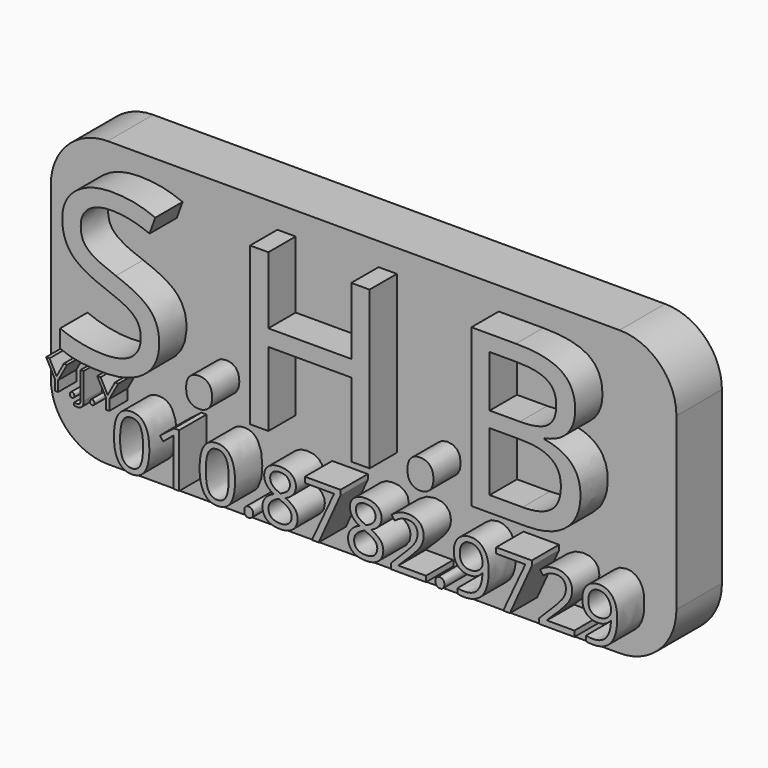
from build123d import *

# Parameters (mm, degrees)
F1_TEXT_SIZE   = 19.38170347
F1_TEXT_SIZE_2 = 6.5863196652
F2_DEPTH       = 8
F0_W           = 55
F0_H           = 25
F3_DEPTH       = 5
F4_R           = 5
F5_TEXT_SIZE   = 3.3051202384
F6_DEPTH       = 2


# Not quite as in the source:
# - Text() gives the source's letters only with a copy of the font that has no kerning and outlines rounded to 1/6400 em; it was checked with that copy


with BuildPart() as f2:
    # F1 (on face) → F2 (new body)
    with BuildSketch(Plane.XZ):
        with Locations((2.2213128849, 9.1533623248)):
            Text('S.H.B', F1_TEXT_SIZE, font='Open Sans', text_align=(TextAlign.LEFT, TextAlign.BOTTOM))
        with Locations((7.6230826626, 1.9649819029)):
            Text('010.8782.9729', F1_TEXT_SIZE_2, font='Open Sans', text_align=(TextAlign.LEFT, TextAlign.BOTTOM))
    extrude(amount=F2_DEPTH)


with BuildPart() as f3:
    # F0 (on Front) → F3 (new body)
    with BuildSketch(Plane.XZ):
        with Locations((27.5, 12.5)):
            Rectangle(F0_W, F0_H)
    extrude(amount=F3_DEPTH)

    # F4
    f4_edges = [f3.edges().sort_by_distance(p)[0] for p in [
        (55, -2.5, 25),
        (0, -2.5, 25),
        (0, -2.5, 0),
        (55, -2.5, 0),
    ]]
    fillet(f4_edges, radius=F4_R)

    # F5 (on face) → F6 (join)
    with BuildSketch(Plane.XZ.offset(5)):
        with Locations((1.1851047166, 5.4952464998)):
            Text('Y.J.Y', F5_TEXT_SIZE, font='Open Sans', text_align=(TextAlign.LEFT, TextAlign.BOTTOM))
    extrude(amount=F6_DEPTH)


solid = Compound([f2.part, f3.part])
